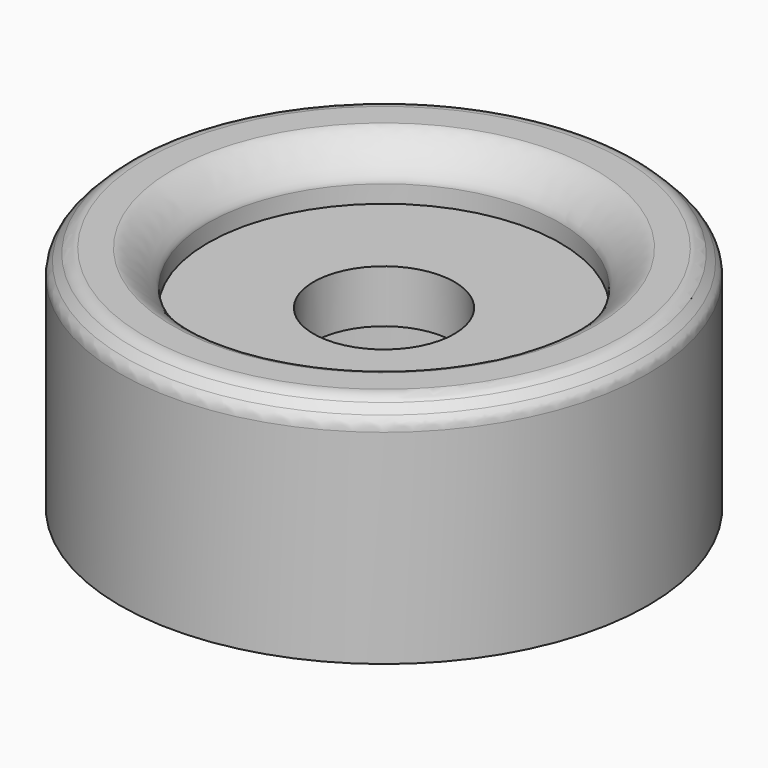
from build123d import *

# Parameters (mm, degrees)
F2_R     = 4
F3_DEPTH = 25
F5_SIZE  = 1
F6_R     = 1


# Not quite as in the source:
# - a fillet or chamfer that OpenCascade refuses, or shapes differently, is made with other operations: its cross-section is extruded or revolved along the edge and cut away or added


with BuildPart() as f1:
    # F0 (on Front) → F1 (revolve)
    with BuildSketch(Plane.XZ):
        Polygon((-10, 0), (0, 0), (0, 3), (-10, 3), (-10, 6), (-15, 6), (-15, -7), (-10, -7), align=None)
    revolve(axis=Axis((0, 0, 1.5), (0, 0, -1)))

    # F2 (on face) → F3 (cut)
    with BuildSketch(Plane.XY.offset(3)):
        Circle(F2_R)
    extrude(amount=-F3_DEPTH, mode=Mode.SUBTRACT)

    # F4: fillet of radius 2 on 1 edges, made by hand

    # F4_s1 → F4_t2 (revolve, cut)
    with BuildSketch(Plane.XZ):
        with BuildLine():
            add(Edge.make_bspline(
                [(-10, 4), (-10, 6), (-12, 6)],
                knots=[0, 0, 0, 1, 1, 1], degree=2, weights=[1, 0.25, 1]))
            Line((-12, 6), (-10, 6))
            Line((-10, 6), (-10, 4))
        make_face()
    revolve(axis=Axis((0, 0, 6), (0, 0, -1)), mode=Mode.SUBTRACT)

    # F5
    f5_edges = [f1.edges().sort_by_distance(p)[0] for p in [
        (15, 0, 6),
    ]]
    chamfer(f5_edges, length=F5_SIZE)

    # F6
    f6_edges = [f1.edges().sort_by_distance(p)[0] for p in [
        (14, 0, 6),
    ]]
    fillet(f6_edges, radius=F6_R)

    # F7: fillet of radius 1 on 1 edges, made by hand

    # F7_s1 → F7_t2 (revolve, cut)
    with BuildSketch(Plane.XZ):
        with BuildLine():
            add(Edge.make_bspline(
                [(-14.7071067812, 5.2928932188), (-15, 5), (-15, 4.5857864376)],
                knots=[0, 0, 0, 1, 1, 1], degree=2, weights=[1, 1, 1]))
            Line((-15, 4.5857864376), (-15, 5))
            Line((-15, 5), (-14.7071067812, 5.2928932188))
        make_face()
    revolve(axis=Axis((0, 0, 5), (0, 0, -1)), mode=Mode.SUBTRACT)


solid = f1.part
